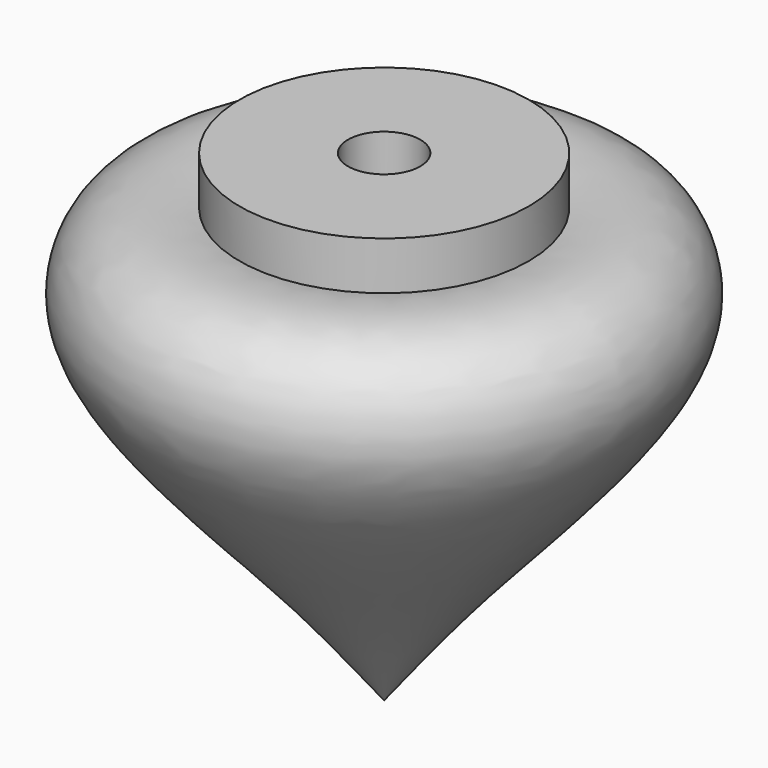
from build123d import *

# Parameters (mm, degrees)
F2_R     = 4.7625
F3_DEPTH = 9.525


# Not quite as in the source:
# - the program builds the solid bodies; features that only make, move or delete a surface that nothing else refers to are left out


with BuildPart() as f1:
    # F0 (on Front) → F1 (revolve)
    with BuildSketch(Plane.XZ):
        with BuildLine():
            Line((19.05, 63.5), (0, 63.5))
            Line((0, 63.5), (0, 0))
            add(Edge.make_bspline(
                [(0, 0), (4.8399250954, 6.2011531554), (11.9044456396, 15.2520698758), (32.1959144321, 36.2100978246), (36.9145185343, 50.2245718319), (29.3633082779, 59.1419363718), (19.05, 57.15)],
                knots=[0, 0, 0, 0, 0.2581105042, 0.5601984274, 0.7643398405, 1, 1, 1, 1], degree=3))
            Line((19.05, 57.15), (19.05, 63.5))
        make_face()
    revolve(axis=Axis((0, 0, 31.75), (0, 0, -1)))

    # F2 (on face) → F3 (cut)
    with BuildSketch(Plane.XY.offset(63.5)):
        Circle(F2_R)
    extrude(amount=-F3_DEPTH, mode=Mode.SUBTRACT)


solid = f1.part
